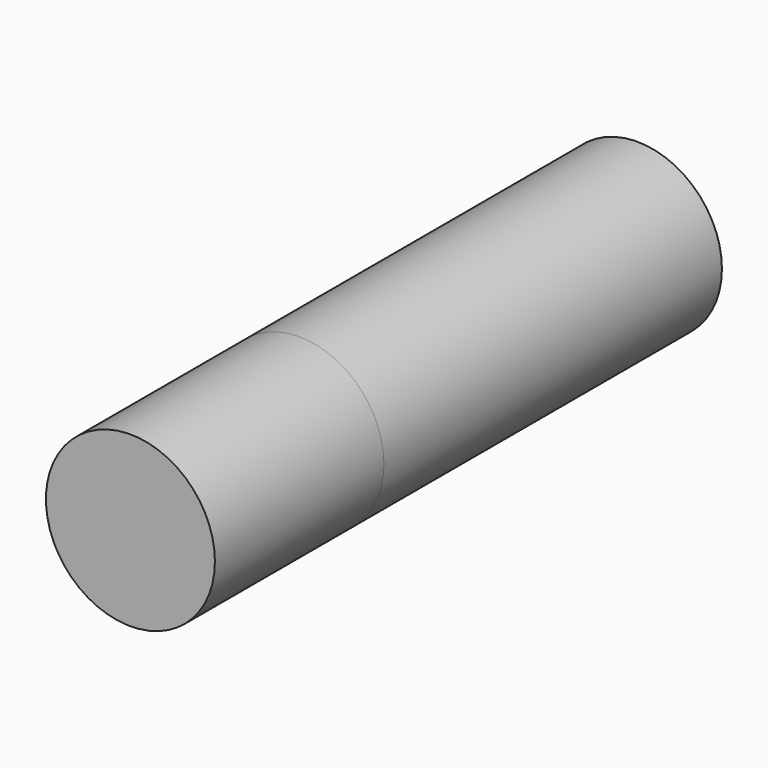
from build123d import *

# Parameters (mm, degrees)
F0_R     = 200
F1_DEPTH = 1000
F2_R     = 200
F3_DEPTH = 500


# Not quite as in the source:
# - a feature names something its author has since deleted; it is built from what else it names


with BuildPart() as f1:
    # F0 (on Front) → F1 (new body)
    with BuildSketch(Plane.XZ):
        with Locations((3.8924142718, -4.3196221814)):
            Circle(F0_R)
    extrude(amount=F1_DEPTH)


with BuildPart() as f3:
    # F2 (on face) → F3 (new body)
    with BuildSketch(Plane.XZ.offset(1000)):
        with Locations((3.8924142718, -4.3196221814)):
            Circle(F2_R)
    extrude(amount=F3_DEPTH)


solid = Compound([f1.part, f3.part])
